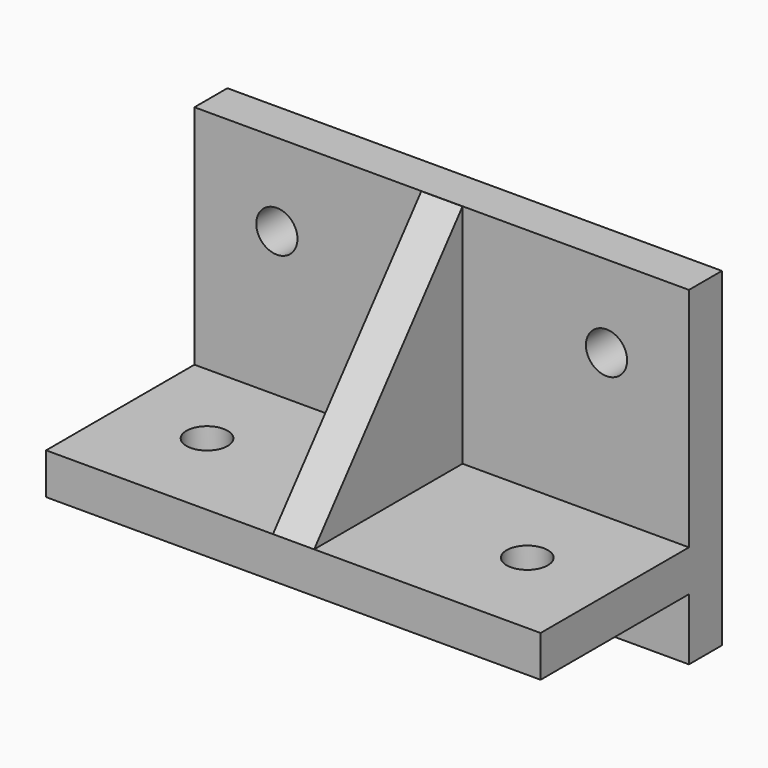
from build123d import *

# Parameters (mm, degrees)
F0_W     = 120
F0_H     = 80
F0_R     = 5
F1_DEPTH = 10
F2_W     = 120
F2_H     = 10
F3_DEPTH = 45
F4_R     = 5
F5_DEPTH = 25
F6_W     = 10
F6_H     = 54.9613343179
F7_DEPTH = 45
F9_DEPTH = 25


# Not quite as in the source:
# - a feature names something its author has since deleted; it is built from what else it names


with BuildPart() as f1:
    # F0 (on Front) → F1 (new body)
    with BuildSketch(Plane.XZ):
        Rectangle(F0_W, F0_H)
        with Locations((-40, 20)):
            Circle(F0_R, mode=Mode.SUBTRACT)
        with Locations((40, 20.0739782304)):
            Circle(F0_R, mode=Mode.SUBTRACT)
    extrude(amount=F1_DEPTH)

    # F2 (on face) → F3 (join)
    with BuildSketch(Plane.XZ.offset(10)):
        with Locations((0, -20)):
            Rectangle(F2_W, F2_H)
    extrude(amount=F3_DEPTH)

    # F4 (on face) → F5 (cut)
    with BuildSketch(Plane.XY.offset(-15)):
        with Locations((-39.2463095486, -32.116651535)):
            Circle(F4_R)
        with Locations((38.7271312058, -32.4570691816)):
            Circle(F4_R)
    extrude(amount=-F5_DEPTH, mode=Mode.SUBTRACT)

    # F6 (on face) → F7 (join)
    with BuildSketch(Plane.XZ.offset(10)):
        with Locations((0.0515476614, 12.480667159)):
            Rectangle(F6_W, F6_H)
    extrude(amount=F7_DEPTH)

    # F8 (on face) → F9 (cut)
    with BuildSketch(Plane(origin=(-4.9484523386, 0, 0), x_dir=(0, -1, 0), z_dir=(-1, 0, 0))):
        Polygon((55, 39.9613343179), (10, 39.9613343179), (55, -15), align=None)
    extrude(amount=-F9_DEPTH, mode=Mode.SUBTRACT)


solid = f1.part
